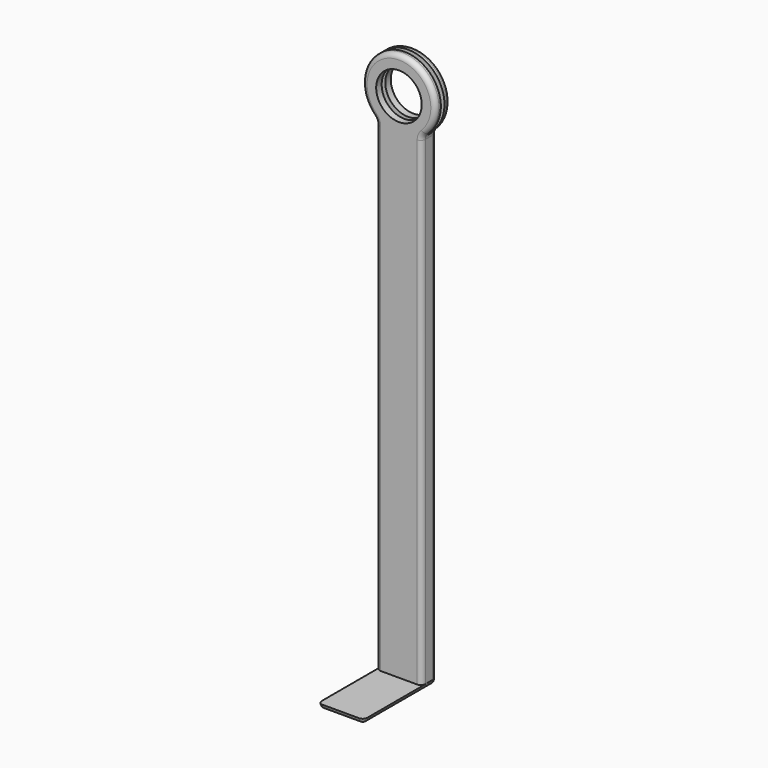
from build123d import *

# Parameters (mm, degrees)
F0_R        = 25
F1_DEPTH    = 20
F3_DEPTH    = 70
F4_R        = 5
F6_DEPTH    = 25
F7_T1_DEPTH = 17.5
F7_T3_DEPTH = 30
F8_R        = 4.99999


# Not quite as in the source:
# - a fillet or chamfer that OpenCascade refuses, or shapes differently, is made with other operations: its cross-section is extruded or revolved along the edge and cut away or added
# - a fillet or chamfer is up to 0.001 mm smaller than in the source, because OpenCascade refuses the exact size


with BuildPart() as f1:
    # F0 (on Front) → F1 (new body)
    with BuildSketch(Plane.XZ):
        with BuildLine():
            Line((-25.1910626888, 440.0464960357), (-25.1910626888, -86.4124843018))
            Line((-25.1910626888, -86.4124843018), (24.8089373112, -86.4124843018))
            Line((24.8089373112, -86.4124843018), (24.8089373112, 440.0464960357))
            ThreePointArc((24.8089373112, 440.0464960357), (25.5893928539, 443.9194793819), (27.8089373112, 447.1879244642))
            ThreePointArc((27.8089373112, 447.1879244642), (-0.1910626888, 515.7536381784), (-28.1910626888, 447.1879244642))
            ThreePointArc((-28.1910626888, 447.1879244642), (-25.9715182315, 443.9194793819), (-25.1910626888, 440.0464960357))
        make_face()
        with Locations((-0.1910626888, 475.7536381784)):
            Circle(F0_R, mode=Mode.SUBTRACT)
    extrude(amount=F1_DEPTH)

    # F2 (on face) → F3 (cut, symmetric)
    with BuildSketch(Plane(origin=(-25.1910626888, 0, 0), x_dir=(0, -1, 0), z_dir=(-1, 0, 0))):
        Polygon((12.5, 447.1879244642), (12.5, 450.7536381784), (12.5, 515.7536381784), (7.5, 515.7536381784), (7.5, 450.7536381784), (7.5, 447.1879244642), (7.5, 443.61721025), (12.5, 443.61721025), align=None)
    extrude(amount=F3_DEPTH, both=True, mode=Mode.SUBTRACT)

    # F4
    f4_edges = [f1.edges().sort_by_distance(p)[0] for p in [
        (-25.191063, -20, 176.817006),
        (-25.191063, 0, 176.817006),
    ]]
    fillet(f4_edges, radius=F4_R)

    # F5 (on Right) → F6 (join, symmetric)
    with BuildSketch(Plane.YZ):
        Polygon((0, -91.4124843018), (0, -86.4124843018), (-20, -86.4124843018), (-100, -86.4124843018), (-100, -91.4124843018), align=None)
    extrude(amount=F6_DEPTH, both=True)

    # F7: fillet of radius 5 on 4 edges, made by hand

    # F7_s2 → F7_t1 (cut)
    with BuildSketch(Plane.XY.offset(-103.9124843018)):
        with BuildLine():
            ThreePointArc((-20, 0), (-23.5355339059, -1.4644660941), (-25, -5))
            Line((-25, -5), (-25, 0))
            Line((-25, 0), (-20, 0))
        make_face()
    extrude(amount=F7_T1_DEPTH, mode=Mode.SUBTRACT)

    # F7_s4 → F7_t3 (cut)
    with BuildSketch(Plane.XY.offset(-103.9124843018)):
        with BuildLine():
            ThreePointArc((20, 0), (23.5355339059, -1.4644660941), (25, -5))
            Line((25, -5), (25, 0))
            Line((25, 0), (20, 0))
        make_face()
        with BuildLine():
            ThreePointArc((-20, -100), (-23.5355339059, -98.5355339059), (-25, -95))
            Line((-25, -95), (-25, -100))
            Line((-25, -100), (-20, -100))
        make_face()
        with BuildLine():
            ThreePointArc((25, -95), (23.5355339059, -98.5355339059), (20, -100))
            Line((20, -100), (25, -100))
            Line((25, -100), (25, -95))
        make_face()
    extrude(amount=F7_T3_DEPTH, mode=Mode.SUBTRACT)

    # F8 (radius 5 in the source; OpenCascade refuses exactly that, so slightly less here)
    f8_edges = [f1.edges().sort_by_distance(p)[0] for p in [
        (23.535534, -98.535534, -91.412484),
        (25, -50, -91.412484),
        (23.535534, -1.464466, -91.412484),
        (0, 0, -91.412484),
        (-23.535534, -1.464466, -91.412484),
        (-25, -50, -91.412484),
        (-23.535534, -98.535534, -91.412484),
        (0, -100, -91.412484),
    ]]
    fillet(f8_edges, radius=F8_R)


solid = f1.part
